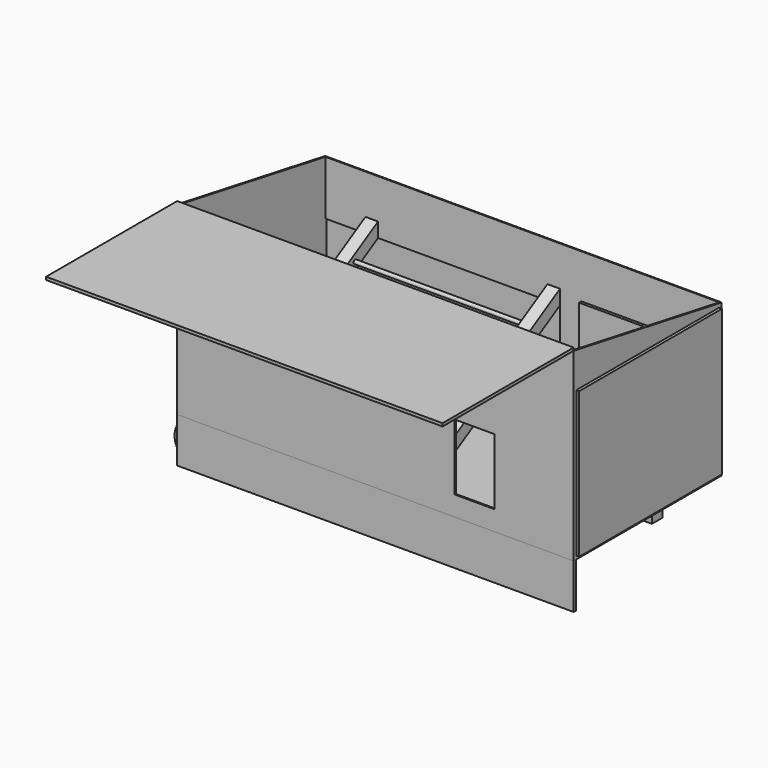
from build123d import *

# Parameters (mm, degrees)
F5_W      = 3000
F5_H      = 1400
F6_DEPTH  = 1400
F7_T      = -10
F10_DEPTH = 3000.001
F11_W     = 22
F11_H     = 340
F11_H_2   = 22
F11_W_2   = 679
F11_H_3   = 350
F11_H_4   = 530.6315167163
F12_DEPTH = 500
F13_W     = 1300
F13_H     = 1053.1422270081
F14_DEPTH = 25
F15_W     = 1350
F15_H     = 1103.1422270081
F16_DEPTH = 22
F19_DEPTH = 95
F21_R     = 15
F22_DEPTH = 1282
F23_W     = 300
F23_H     = 500
F24_DEPTH = 25
F25_W     = 1240
F25_H     = 22
F26_DEPTH = 3000
F27_W     = 1775
F27_H     = 733.4456758621
F28_DEPTH = 25
F29_W     = 1810
F29_H     = 768.4456758621
F30_DEPTH = 22
F31_W     = 3000
F31_H     = 22
F32_DEPTH = 340
F33_W     = 101.2148975914
F33_H     = 101.2148975914
F34_DEPTH = 340
F36_R     = 160
F36_R_2   = 10
F37_DEPTH = 95
F38_W     = 300
F38_H     = 95
F39_DEPTH = 190
F41_DEPTH = 1480.001
F42_W     = 100
F42_H     = 40
F43_DEPTH = 5
F45_R     = 10
F46_DEPTH = 1300


# Not quite as in the source:
# - a feature of the source that left no trace in its solid (it failed there, or was rolled back) is left out
# - a pattern or mirror of a feature is missing from the dataset's text; its kind, count and spacing are read off the source's solid


with BuildPart() as f6:
    # F5 (on offset) → F6 (new body)
    with BuildSketch(Plane.XY.offset(340)):
        Rectangle(F5_W, F5_H)
    extrude(amount=F6_DEPTH)

    # F7
    f7_openings = [f6.faces().sort_by_distance(p)[0] for p in [
        (0, 0, 1740),
    ]]
    offset(amount=F7_T, openings=f7_openings)

    # F9 (on face) → F10 (cut, through all)
    with BuildSketch(Plane(origin=(-1500, 0, 0), x_dir=(0, -1, 0), z_dir=(-1, 0, 0))):
        Polygon((-923.6419556025, 1453.708116217), (851.2289943782, 1766.6657519743), (692.6008882609, 2226.9985032484), (-1018.4111959435, 1991.1711860221), align=None)
    extrude(amount=-F10_DEPTH, mode=Mode.SUBTRACT)

    # F13 (on face) → F14 (cut)
    with BuildSketch(Plane.YZ.offset(1500)):
        with Locations((0, 916.5711135041)):
            Rectangle(F13_W, F13_H)
    extrude(amount=-F14_DEPTH, mode=Mode.SUBTRACT)

    # F23 (on face) → F24 (cut)
    with BuildSketch(Plane.XZ.offset(700)):
        with Locations((750, 740)):
            Rectangle(F23_W, F23_H)
    extrude(amount=-F24_DEPTH, mode=Mode.SUBTRACT)

    # F27 (on face) → F28 (cut)
    with BuildSketch(Plane(origin=(0, 700, 0), x_dir=(-1, 0, 0), z_dir=(0, 1, 0))):
        with Locations((602.5, 716.7228379311)):
            Rectangle(F27_W, F27_H)
    extrude(amount=-F28_DEPTH, mode=Mode.SUBTRACT)


with BuildPart() as f12:
    # F11 (on face) → F12 (new body)
    with BuildSketch(Plane(origin=(1490, 0, 0), x_dir=(0, -1, 0), z_dir=(-1, 0, 0))):
        with Locations((0, 520)):
            Rectangle(F11_W, F11_H)
        with Locations((0, 701)):
            Rectangle(F11_W, F11_H_2)
        with Locations((350.5, 701)):
            Rectangle(F11_W_2, F11_H_2)
        with Locations((-350.5, 701)):
            Rectangle(F11_W_2, F11_H_2)
        with Locations((0, 887)):
            Rectangle(F11_W, F11_H_3)
        with Locations((0, 1073)):
            Rectangle(F11_W, F11_H_2)
        with Locations((350.5, 1073)):
            Rectangle(F11_W_2, F11_H_2)
        with Locations((-350.5, 1073)):
            Rectangle(F11_W_2, F11_H_2)
        with Locations((0, 1349.3157583581)):
            Rectangle(F11_W, F11_H_4)
    extrude(amount=F12_DEPTH)


with BuildPart() as f16:
    # F15 (on face) → F16 (new body)
    with BuildSketch(Plane.YZ.offset(1500)):
        with Locations((0, 916.5711135041)):
            Rectangle(F15_W, F15_H)
    extrude(amount=F16_DEPTH)


with BuildPart() as f19:
    # F18 (on offset) → F19 (new body)
    with BuildSketch(Plane.YZ.offset(190)):
        Polygon((690, 1083.4456758621), (690, 1193.1422270081), (-454.660094428, 532.2724133595), (-407.160094428, 450), align=None)
    extrude(amount=F19_DEPTH)


with BuildPart() as f19_copies_1:
    # F19_copies: instance of F19
    add(f19.part.mirror(Plane(origin=(-451, 0, 0), x_dir=(0, 0, -1), z_dir=(-1, 0, 0))))


with BuildPart() as f22:
    # F21 (on face) → F22 (new body, through all)
    with BuildSketch(Plane(origin=(190, 0, 0), x_dir=(0, -1, 0), z_dir=(-1, 0, 0))):
        with Locations((-473.4936490539, 1013.2939514351)):
            Circle(F21_R)
    extrude(amount=F22_DEPTH)


with BuildPart() as f22b:
    # F21 (on face) → F22, piece 2 (new body, through all)
    with BuildSketch(Plane(origin=(190, 0, 0), x_dir=(0, -1, 0), z_dir=(-1, 0, 0))):
        with Locations((-213.6860279186, 863.2939514351)):
            Circle(F21_R)
    extrude(amount=F22_DEPTH)


with BuildPart() as f22c:
    # F21 (on face) → F22, piece 3 (new body, through all)
    with BuildSketch(Plane(origin=(190, 0, 0), x_dir=(0, -1, 0), z_dir=(-1, 0, 0))):
        with Locations((46.1215932168, 713.2939514351)):
            Circle(F21_R)
    extrude(amount=F22_DEPTH)


with BuildPart() as f26:
    # F25 (on face) → F26 (new body, through all)
    with BuildSketch(Plane(origin=(-1500, 0, 0), x_dir=(0, -1, 0), z_dir=(-1, 0, 0))):
        with Locations((1320, 1751)):
            Rectangle(F25_W, F25_H)
    extrude(amount=-F26_DEPTH)


with BuildPart() as f30:
    # F29 (on face) → F30 (new body)
    with BuildSketch(Plane(origin=(0, 700, 0), x_dir=(-1, 0, 0), z_dir=(0, 1, 0))):
        with Locations((595, 724.2228379311)):
            Rectangle(F29_W, F29_H)
    extrude(amount=F30_DEPTH)


with BuildPart() as f32:
    # F31 (on face) → F32 (new body)
    with BuildSketch(Plane(origin=(0, 0, 340), x_dir=(1, 0, 0), z_dir=(0, 0, -1))):
        with Locations((0, 689)):
            Rectangle(F31_W, F31_H)
    extrude(amount=F32_DEPTH)


with BuildPart() as f34:
    # F33 (on face) → F34 (new body)
    with BuildSketch(Plane(origin=(0, 0, 340), x_dir=(1, 0, 0), z_dir=(0, 0, -1))):
        with Locations((1105.8368849942, 523.8840551683)):
            Rectangle(F33_W, F33_H)
    extrude(amount=F34_DEPTH)


with BuildPart() as f34b:
    # F33 (on face) → F34, piece 2 (new body)
    with BuildSketch(Plane(origin=(0, 0, 340), x_dir=(1, 0, 0), z_dir=(0, 0, -1))):
        with Locations((1105.8368849942, -520.4225837978)):
            Rectangle(F33_W, F33_H)
    extrude(amount=F34_DEPTH)


with BuildPart() as f37:
    # F36 (on offset) → F37 (new body)
    with BuildSketch(Plane.XZ.offset(650)):
        with Locations((-1400, 160)):
            Circle(F36_R)
        with Locations((-1400, 160)):
            Circle(F36_R_2, mode=Mode.SUBTRACT)
    extrude(amount=-F37_DEPTH)


with BuildPart() as f39:
    # F38 (on face) → F39 (new body)
    with BuildSketch(Plane(origin=(0, 0, 340), x_dir=(1, 0, 0), z_dir=(0, 0, -1))):
        with Locations((-1350, 507.5)):
            Rectangle(F38_W, F38_H)
    extrude(amount=F39_DEPTH)

    # F40 (on face) → F41 (cut, through all)
    with BuildSketch(Plane(origin=(0, -460, 0), x_dir=(-1, 0, 0), z_dir=(0, 1, 0))):
        with BuildLine():
            Line((1410, 150), (1410, 160))
            ThreePointArc((1410, 160), (1400, 170), (1390, 160))
            Line((1390, 160), (1390, 150))
            Line((1390, 150), (1410, 150))
        make_face()
    extrude(amount=-F41_DEPTH, mode=Mode.SUBTRACT)


with BuildPart() as f43:
    # F42 (on face) → F43 (new body)
    with BuildSketch(Plane(origin=(0, 0, 150), x_dir=(1, 0, 0), z_dir=(0, 0, -1))):
        with Locations((-1400, 480)):
            Rectangle(F42_W, F42_H)
    extrude(amount=F43_DEPTH)


with BuildPart() as f43b:
    # F42 (on face) → F43, piece 2 (new body)
    with BuildSketch(Plane(origin=(0, 0, 150), x_dir=(1, 0, 0), z_dir=(0, 0, -1))):
        with Locations((-1400, 535)):
            Rectangle(F42_W, F42_H)
    extrude(amount=F43_DEPTH)


with BuildPart() as f44_1:
    # F44: instance of F37
    add(f37.part.mirror(Plane.XZ))


with BuildPart() as f44_2:
    # F44: instance of F39
    add(f39.part.mirror(Plane.XZ))


with BuildPart() as f44_3:
    # F44: instance of F43b
    add(f43b.part.mirror(Plane.XZ))


with BuildPart() as f44_4:
    # F44: instance of F43
    add(f43.part.mirror(Plane.XZ))


with BuildPart() as f46:
    # F45 (on face) → F46 (new body, through all)
    with BuildSketch(Plane(origin=(0, 650, 0), x_dir=(-1, 0, 0), z_dir=(0, 1, 0))):
        with Locations((1400, 160)):
            Circle(F45_R)
    extrude(amount=-F46_DEPTH)


solid = Compound([f6.part, f12.part, f16.part, f19.part, f19_copies_1.part, f22.part, f22b.part, f22c.part, f26.part, f30.part, f32.part, f34.part, f34b.part, f37.part, f39.part, f43.part, f43b.part, f44_1.part, f44_2.part, f44_3.part, f44_4.part, f46.part])
